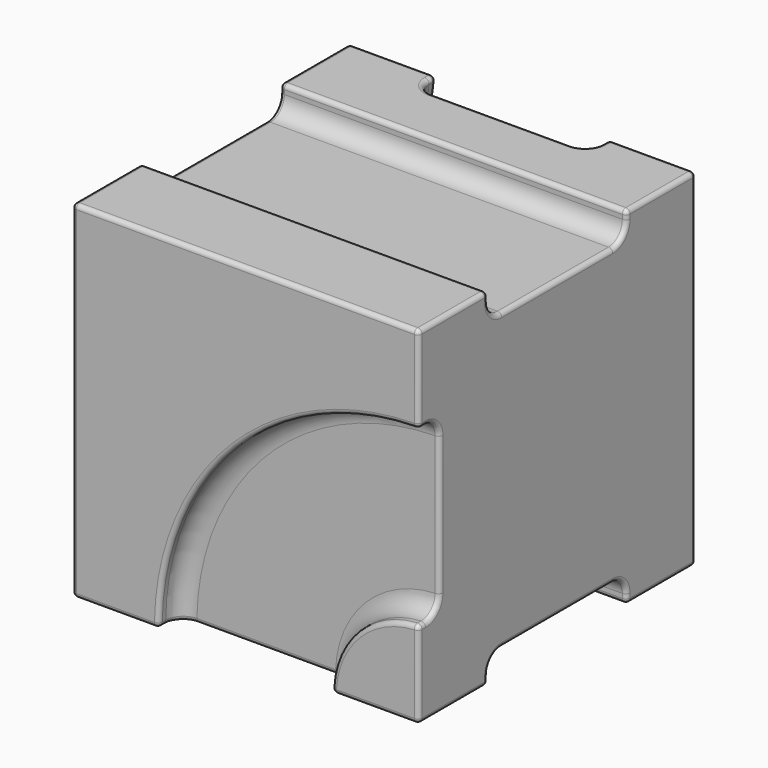
from build123d import *

# Parameters (mm, degrees)
F0_W     = 40
F0_H     = 40
F1_DEPTH = 20
F3_DEPTH = 3
F4_W     = 40
F4_H     = 20
F5_DEPTH = 3
F7_DEPTH = 3
F9_DEPTH = 3
F10_R    = 2
F11_R    = 0.5


# Not quite as in the source:
# - a feature names something its author has since deleted; it is built from what else it names


with BuildPart() as f1:
    # F0 (on Front) → F1 (new body, symmetric)
    with BuildSketch(Plane.XZ):
        Rectangle(F0_W, F0_H)
    extrude(amount=F1_DEPTH, both=True)

    # F2 (on face) → F3 (cut)
    with BuildSketch(Plane.XY.offset(20)):
        Polygon((20, 0), (20, 10), (-20, 10), (-20, 0), (-20, -10), (20, -10), align=None)
    extrude(amount=-F3_DEPTH, mode=Mode.SUBTRACT)

    # F4 (on face) → F5 (cut)
    with BuildSketch(Plane(origin=(0, 0, -20), x_dir=(1, 0, 0), z_dir=(0, 0, -1))):
        Rectangle(F4_W, F4_H)
    extrude(amount=-F5_DEPTH, mode=Mode.SUBTRACT)

    # F6 (on face) → F7 (cut)
    with BuildSketch(Plane.XZ.offset(20)):
        with BuildLine():
            Line((-10, -20), (10, -20))
            ThreePointArc((10, -20), (12.9289321881, -12.9289321881), (20, -10))
            Line((20, -10), (20, 10))
            ThreePointArc((20, 10), (-1.2132034356, 1.2132034356), (-10, -20))
        make_face()
    extrude(amount=-F7_DEPTH, mode=Mode.SUBTRACT)

    # F8 (on face) → F9 (cut)
    with BuildSketch(Plane(origin=(0, 20, 0), x_dir=(-1, 0, 0), z_dir=(0, 1, 0))):
        with BuildLine():
            Line((20, -10), (20, 10))
            ThreePointArc((20, 10), (12.9289321881, 12.9289321881), (10, 20))
            Line((10, 20), (-10, 20))
            ThreePointArc((-10, 20), (-1.2132034356, -1.2132034356), (20, -10))
        make_face()
        with BuildLine():
            ThreePointArc((10, -20), (12.9289321881, -12.9289321881), (20, -10))
            ThreePointArc((20, -10), (-1.2132034356, -1.2132034356), (-10, 20))
            Line((-10, 20), (-10, -20))
            Line((-10, -20), (10, -20))
        make_face()
    extrude(amount=-F9_DEPTH, mode=Mode.SUBTRACT)

    # F10
    f10_edges = [f1.edges().sort_by_distance(p)[0] for p in [
        (0, 10, -17),
        (0, -10, -17),
        (-1.213203, -17, 1.213203),
        (12.928932, -17, -12.928932),
        (10, 17, 0),
        (-12.928932, 17, 12.928932),
        (-12.928932, 17, -12.928932),
        (0, -10, 17),
        (0, 10, 17),
    ]]
    fillet(f10_edges, radius=F10_R)

    # F11
    f11_edges = [f1.edges().sort_by_distance(p)[0] for p in [
        (12.928932, -20, -12.928932),
        (20, -20, -15),
        (15, -20, -20),
        (-20, -20, 0),
        (0, -20, 20),
        (20, -20, 15),
        (-1.213203, -20, 1.213203),
        (-15, -20, -20),
        (-20, 10, 19.5),
        (-20, 9.414214, 17.585786),
        (-20, 15, 20),
        (-20, 0, 17),
        (-20, 20, 15),
        (-20, -9.414214, 17.585786),
        (-20, 19.5, 10),
        (-20, -10, 19.5),
        (-20, 17.585786, 9.414214),
        (-20, -15, 20),
        (-20, 17, 0),
        (-20, 17.585786, -9.414214),
        (-20, -15, -20),
        (-20, 19.5, -10),
        (-20, -10, -19.5),
        (-20, 20, -15),
        (-20, -9.414214, -17.585786),
        (-20, 15, -20),
        (-20, 0, -17),
        (-20, 10, -19.5),
        (-20, 9.414214, -17.585786),
        (-10, -19.5, -20),
        (-9.414214, -17.585786, -20),
        (0, -17, -20),
        (9.414214, -17.585786, -20),
        (0, -10, -20),
        (10, -19.5, -20),
        (20, -15, -20),
        (10, 19.5, -20),
        (9.414214, 17.585786, -20),
        (15, 20, -20),
        (0, 17, -20),
        (20, 15, -20),
        (-9.414214, 17.585786, -20),
        (0, 10, -20),
        (-10, 19.5, -20),
        (-15, 20, -20),
        (10, 20, 0),
        (15, 20, 20),
        (20, 20, 0),
        (-12.928932, 20, -12.928932),
        (-15, 20, 20),
        (-12.928932, 20, 12.928932),
        (20, 10, -19.5),
        (20, 9.414214, -17.585786),
        (20, 0, -17),
        (20, -9.414214, -17.585786),
        (20, 15, 20),
        (20, -10, -19.5),
        (20, 10, 19.5),
        (20, 9.414214, 17.585786),
        (20, 0, 17),
        (20, -19.5, -10),
        (20, -9.414214, 17.585786),
        (20, -17.585786, -9.414214),
        (20, -10, 19.5),
        (20, -17, 0),
        (20, -15, 20),
        (20, -17.585786, 9.414214),
        (20, -19.5, 10),
        (-10, 19.5, 20),
        (-9.414214, 17.585786, 20),
        (0, 17, 20),
        (9.414214, 17.585786, 20),
        (0, 10, 20),
        (10, 19.5, 20),
        (0, -10, 20),
    ]]
    fillet(f11_edges, radius=F11_R)


solid = f1.part
